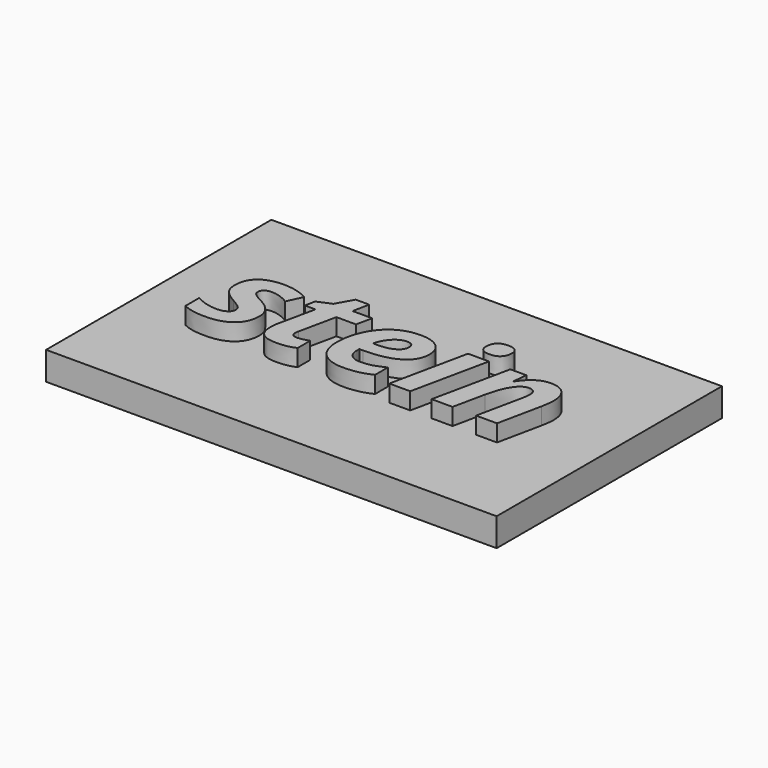
from build123d import *

# Parameters (mm, degrees)
F0_W         = 80
F0_H         = 50
F1_DEPTH     = 5
F2_TEXT_SIZE = 25.3078501879
F3_DEPTH     = 3


# Not quite as in the source:
# - Text() gives the source's letters only with a copy of the font that has no kerning and outlines rounded to 1/6400 em; it was checked with that copy


with BuildPart() as f1:
    # F0 (on Top) → F1 (new body)
    with BuildSketch(Plane.XY):
        with Locations((40, 25)):
            Rectangle(F0_W, F0_H)
    extrude(amount=F1_DEPTH)

    # F2 (on face) → F3 (join)
    with BuildSketch(Plane.XY.offset(5)):
        with Locations((10.1675251499, 17.3195879906)):
            Text('stein', F2_TEXT_SIZE, font='Open Sans', font_style=FontStyle.BOLDITALIC, text_align=(TextAlign.LEFT, TextAlign.BOTTOM))
    extrude(amount=F3_DEPTH)


solid = f1.part
